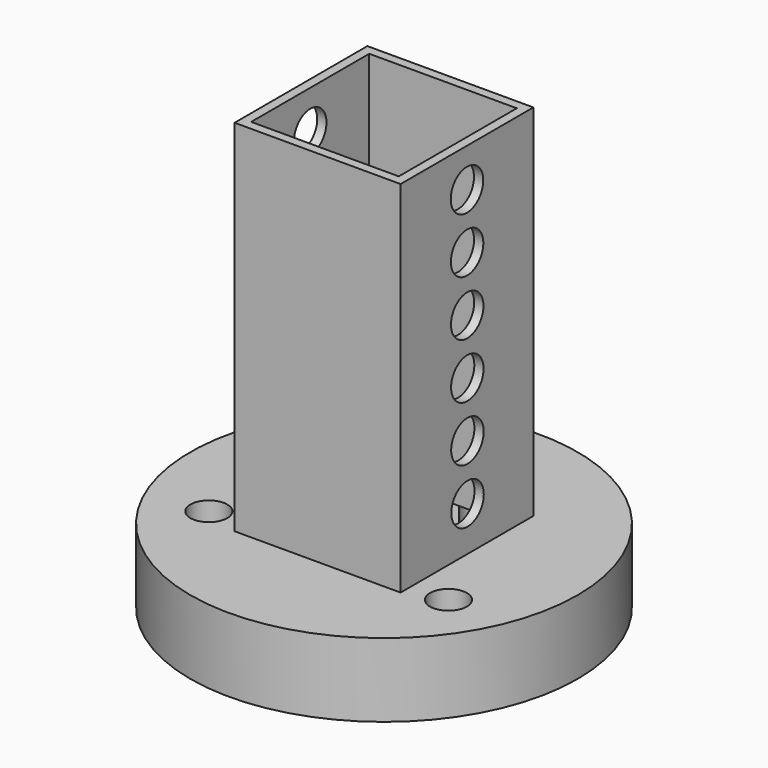
from build123d import *

# Parameters (mm, degrees)
F0_R     = 50
F0_R_2   = 7.5
F1_DEPTH = 15
F2_W     = 40
F2_H     = 40
F3_DEPTH = 100
F4_T     = 2.5
F5_R     = 5.5
F6_DEPTH = 42.5


# Not quite as in the source:
# - a pattern or mirror of a feature is missing from the dataset's text; its kind, count and spacing are read off the source's solid


with BuildPart() as f1:
    # F0 (on Top) → F1 (new body)
    with BuildSketch(Plane.XY):
        Circle(F0_R)
        with Locations((-32.4759526419, -18.75)):
            Circle(F0_R_2, mode=Mode.SUBTRACT)
        with Locations((32.4759526419, -18.75)):
            Circle(F0_R_2, mode=Mode.SUBTRACT)
        with Locations((0, 37.5)):
            Circle(F0_R_2, mode=Mode.SUBTRACT)
    extrude(amount=F1_DEPTH)

    # F2 (on face) → F3 (join)
    with BuildSketch(Plane.XY.offset(15)):
        Rectangle(F2_W, F2_H)
    extrude(amount=F3_DEPTH)

    # F4
    f4_openings = [f1.faces().sort_by_distance(p)[0] for p in [
        (0, 0, 115),
    ]]
    offset(amount=F4_T, openings=f4_openings, kind=Kind.INTERSECTION)

    # F5 (on face) → F6 (cut, through all)
    with BuildSketch(Plane.YZ.offset(22.5)):
        with Locations((0, 104.5)):
            Circle(F5_R)
        with Locations((0.0376883232, 89.5000473471)):
            Circle(F5_R)
        with Locations((0.0753766465, 74.5000946941)):
            Circle(F5_R)
        with Locations((0.1130649697, 59.5001420412)):
            Circle(F5_R)
        with Locations((0.150753293, 44.5001893883)):
            Circle(F5_R)
        with Locations((0.1884416162, 29.5002367353)):
            Circle(F5_R)
    f6 = extrude(amount=-F6_DEPTH, mode=Mode.SUBTRACT)

    # F6_copies: F6 across plane
    add(f6.mirror(Plane(origin=(0, 0, 0), x_dir=(0, 0, -1), z_dir=(-1, 0, 0))), mode=Mode.SUBTRACT)


solid = f1.part
